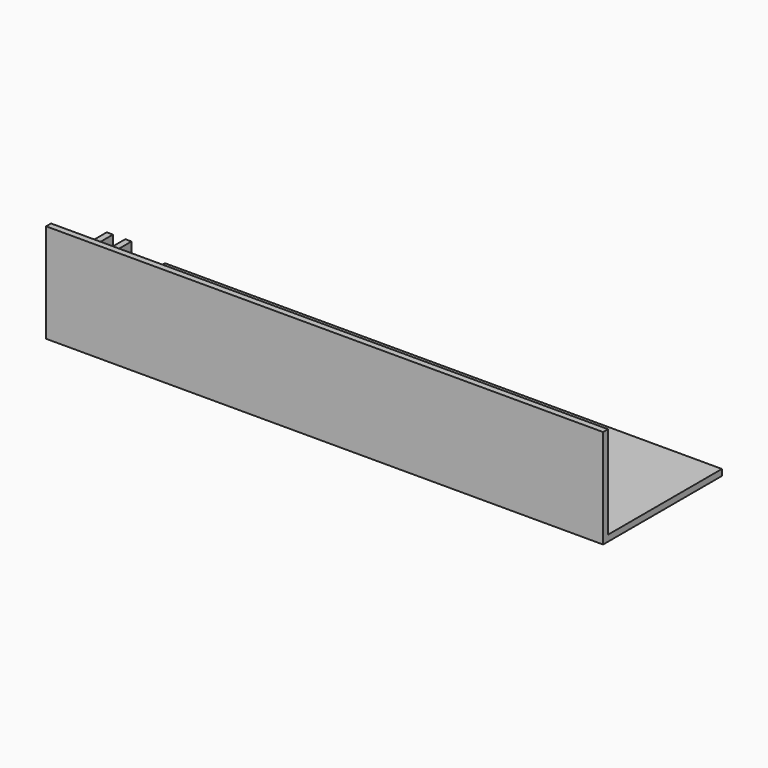
from build123d import *

# Parameters (mm, degrees)
F0_W      = 285.75
F0_H      = 76.2
F1_DEPTH  = 3.175
F2_W      = 285.75
F2_H      = 3.175
F3_DEPTH  = 47.625
F4_W      = 6.35
F4_H      = 25.4
F5_DEPTH  = 25.4
F6_R      = 12.69999
F7_R      = 3.175
F8_DEPTH  = 6.35
F9_R      = 3.175
F10_DEPTH = 3.175
F11_R     = 3.175
F12_DEPTH = 3.175
F13_R     = 3.175
F14_DEPTH = 25.4
F15_R     = 3.175
F16_DEPTH = 25.4
F17_R     = 3.175
F18_DEPTH = 12.7
F20_DEPTH = 6.35


# Not quite as in the source:
# - a fillet or chamfer is up to 0.001 mm smaller than in the source, because OpenCascade refuses the exact size
# - ends of sketch curves that miss each other by under 0.0002 mm in the source are joined


with BuildPart() as f1:
    # F0 (on Top) → F1 (new body)
    with BuildSketch(Plane.XY):
        with Locations((5.1656402647, 2.8847559522)):
            Rectangle(F0_W, F0_H)
    extrude(amount=F1_DEPTH)

    # F2 (on face) → F3 (join)
    with BuildSketch(Plane.XY.offset(3.175)):
        with Locations((5.1656402647, -33.6277440478)):
            Rectangle(F2_W, F2_H)
    extrude(amount=F3_DEPTH)

    # F4 (on face) → F5 (join)
    with BuildSketch(Plane.XY.offset(3.175)):
        with Locations((-128.1843597353, -9.8152440478)):
            Rectangle(F4_W, F4_H)
    extrude(amount=F5_DEPTH)

    # F6 (radius 12.7 in the source; OpenCascade refuses exactly that, so slightly less here)
    f6_edges = [f1.edges().sort_by_distance(p)[0] for p in [
        (-128.18436, 2.884756, 28.575),
        (-128.18436, -22.515244, 28.575),
    ]]
    fillet(f6_edges, radius=F6_R)

    # F7 (on face) → F8 (cut)
    with BuildSketch(Plane(origin=(-131.3593597353, 0, 0), x_dir=(0, -1, 0), z_dir=(-1, 0, 0))):
        with Locations((9.8152440478, 15.875)):
            Circle(F7_R)
    extrude(amount=-F8_DEPTH, mode=Mode.SUBTRACT)


with BuildPart() as f10:
    # F9 (on face) → F10 (new body)
    with BuildSketch(Plane.YZ.offset(-125.0093597353)):
        with BuildLine():
            Line((-19.3402440478, 34.925), (-19.3402440478, 24.275266633))
            ThreePointArc((-19.3402440478, 24.275266633), (-15.0405086236, 27.4502620758), (-9.8152540478, 28.575))
            ThreePointArc((-9.8152540478, 28.575), (-4.589979472, 27.4502620758), (-0.2902440478, 24.275266633))
            Line((-0.2902440478, 24.275266633), (-0.2902440478, 34.925))
            Line((-0.2902440478, 34.925), (-19.3402440478, 34.925))
        make_face()
        with BuildLine():
            Line((-19.3402440478, 24.275266633), (-19.3402440478, 9.525))
            Line((-19.3402440478, 9.525), (-0.2902440478, 9.525))
            Line((-0.2902440478, 9.525), (-0.2902440478, 24.275266633))
            ThreePointArc((-0.2902440478, 24.275266633), (-4.589979472, 27.4502620758), (-9.8152340478, 28.575))
            ThreePointArc((-9.8152340478, 28.575), (-15.0405086236, 27.4502620758), (-19.3402440478, 24.275266633))
        make_face()
        with Locations((-9.8152440478, 15.875)):
            Circle(F9_R, mode=Mode.SUBTRACT)
    extrude(amount=F10_DEPTH)


with BuildPart() as f12:
    # F11 (on face) → F12 (new body)
    with BuildSketch(Plane(origin=(-131.3593597353, 0, 0), x_dir=(0, -1, 0), z_dir=(-1, 0, 0))):
        with BuildLine():
            ThreePointArc((9.8152340478, 28.575), (4.589979472, 27.4502620758), (0.2902440478, 24.275266633))
            Line((0.2902440478, 24.275266633), (0.2902440478, 9.525))
            Line((0.2902440478, 9.525), (19.3402440478, 9.525))
            Line((19.3402440478, 9.525), (19.3402440478, 24.275266633))
            ThreePointArc((19.3402440478, 24.275266633), (15.0405086236, 27.4502620758), (9.8152340478, 28.575))
        make_face()
        with Locations((9.8152440478, 15.875)):
            Circle(F11_R, mode=Mode.SUBTRACT)
        with BuildLine():
            Line((19.3402440478, 34.925), (0.2902440478, 34.925))
            Line((0.2902440478, 34.925), (0.2902440478, 24.275266633))
            ThreePointArc((0.2902440478, 24.275266633), (4.589979472, 27.4502620758), (9.8152340478, 28.575))
            ThreePointArc((9.8152340478, 28.575), (15.0405086236, 27.4502620758), (19.3402440478, 24.275266633))
            Line((19.3402440478, 24.275266633), (19.3402440478, 34.925))
        make_face()
    extrude(amount=F12_DEPTH)


with BuildPart() as f14_tool:
    # F13 (on face) → F14 (new body)
    with BuildSketch(Plane(origin=(-134.5343597353, 0, 0), x_dir=(0, -1, 0), z_dir=(-1, 0, 0))):
        with Locations((9.8152440478, 28.575)):
            Circle(F13_R)
    extrude(amount=-F14_DEPTH)


with BuildPart() as f1_1:
    add(f1.part)

    # F14: cut by f14_tool
    add(f14_tool.part, mode=Mode.SUBTRACT)

    # F15 (on face) → F16 (cut)
    with BuildSketch(Plane.YZ.offset(-121.8343597353)):
        with Locations((-9.8152440478, 28.575)):
            Circle(F15_R)
    extrude(amount=-F16_DEPTH, mode=Mode.SUBTRACT)

    # F19 (on face) → F20 (cut)
    with BuildSketch(Plane(origin=(-131.3593597353, 0, 0), x_dir=(0, -1, 0), z_dir=(-1, 0, 0))):
        with BuildLine():
            ThreePointArc((12.9653419757, 28.1781271679), (12.9840124143, 28.376173343), (12.9902440478, 28.575))
            ThreePointArc((12.9902440478, 28.575), (9.6164173909, 31.7437683665), (6.66514612, 28.1781271679))
            ThreePointArc((6.66514612, 28.1781271679), (9.8152440478, 25.4), (12.9653419757, 28.1781271679))
        make_face()
    extrude(amount=-F20_DEPTH, mode=Mode.SUBTRACT)


with BuildPart() as f10_1:
    add(f10.part)

    # F14: cut by f14_tool
    add(f14_tool.part, mode=Mode.SUBTRACT)


with BuildPart() as f12_1:
    add(f12.part)

    # F14: cut by f14_tool
    add(f14_tool.part, mode=Mode.SUBTRACT)


with BuildPart() as f18:
    # F17 (on face) → F18 (new body)
    with BuildSketch(Plane(origin=(-134.5343597353, 0, 0), x_dir=(0, -1, 0), z_dir=(-1, 0, 0))):
        with Locations((9.8152440478, 15.875)):
            Circle(F17_R)
    extrude(amount=-F18_DEPTH)


solid = Compound([f1_1.part, f10_1.part, f12_1.part, f18.part])
